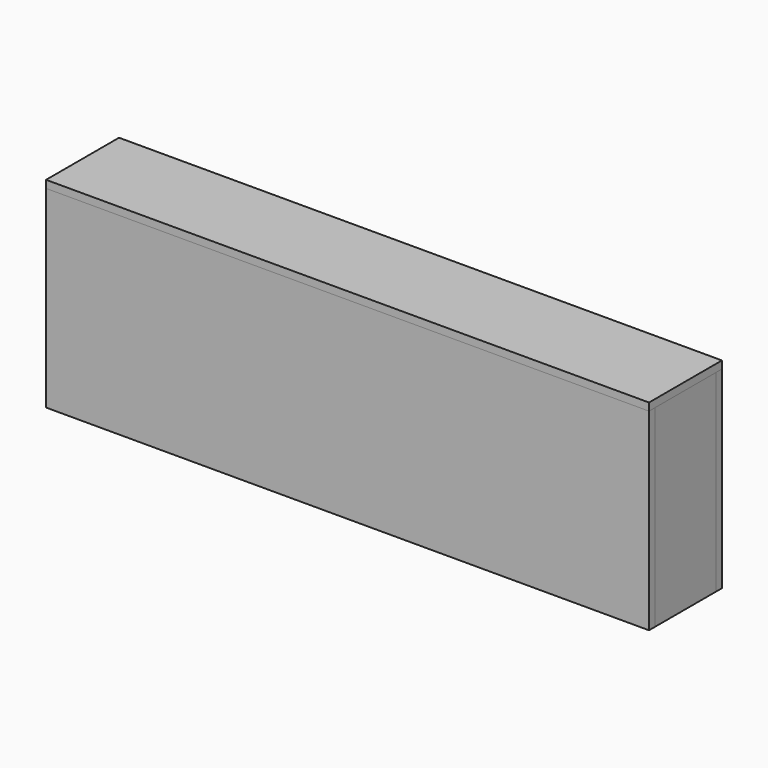
from build123d import *
from build123d import SkipClean  # not in build123d's __all__

# Parameters (mm, degrees)
F1_DEPTH  = 20
F5_R      = 8
F6_DEPTH  = 21.6502592253
F8_W      = 158.75
F8_H      = 50.8
F9_DEPTH  = 2
F10_W     = 158.75
F10_H     = 50.8
F11_DEPTH = 2
F12_W     = 158.75
F12_H     = 24
F13_DEPTH = 2


# Not quite as in the source:
# - a feature names something its author has since deleted; it is built from what else it names


with BuildPart() as f1:
    # F0 (on Front) → F1 (new body)
    with BuildSketch(Plane.XZ):
        with BuildLine():
            Line((18.991692129, -26.1704544329), (18.991692129, -33.7295945078))
            Line((18.991692129, -33.7295945078), (98.366692129, -33.7295945078))
            Line((98.366692129, -33.7295945078), (98.366692129, 17.0704054922))
            Line((98.366692129, 17.0704054922), (85.666692129, 17.0704054922))
            ThreePointArc((85.666692129, 17.0704054922), (58.7262098437, -14.413869844), (18.991692129, -26.1704544329))
        make_face()
    extrude(amount=F1_DEPTH)

    # F5 (on face) → F6 (cut, through all)
    with BuildSketch(Plane(origin=(94.705044452, 0, -6.6224218335), x_dir=(0, 1, 0), z_dir=(0.9975640503, 0, -0.0697564737))):
        with Locations((-10, 11.1905364192)):
            Circle(F5_R)
    extrude(amount=-F6_DEPTH, mode=Mode.SUBTRACT)

    # F7: F1 across face


with BuildPart() as f1_1:
    add(f1.part, clean=False)
    with SkipClean():  # cleaning this boolean's faces spoils the solid; the shape is the same uncleaned
        add(f1.part.mirror(Plane(origin=(18.991692129, -10, -29.9500244704), x_dir=(0, -1, 0), z_dir=(-1, 0, 0))), clean=False)


with BuildPart() as f9:
    # F8 (on face) → F9 (new body)
    with BuildSketch(Plane(origin=(0, 0, 0), x_dir=(-1, 0, 0), z_dir=(0, 1, 0))):
        with Locations((-18.991692129, -8.3295945078)):
            Rectangle(F8_W, F8_H)
    extrude(amount=F9_DEPTH)


with BuildPart() as f11:
    # F10 (on face) → F11 (new body)
    with BuildSketch(Plane.XZ.offset(20)):
        with Locations((18.991692129, -8.3295945078)):
            Rectangle(F10_W, F10_H)
    extrude(amount=F11_DEPTH)


with BuildPart() as f13:
    # F12 (on face) → F13 (new body)
    with BuildSketch(Plane.XY.offset(17.0704054922)):
        with Locations((18.991692129, -10)):
            Rectangle(F12_W, F12_H)
    extrude(amount=F13_DEPTH)


solid = Compound([f1_1.part, f9.part, f11.part, f13.part])
